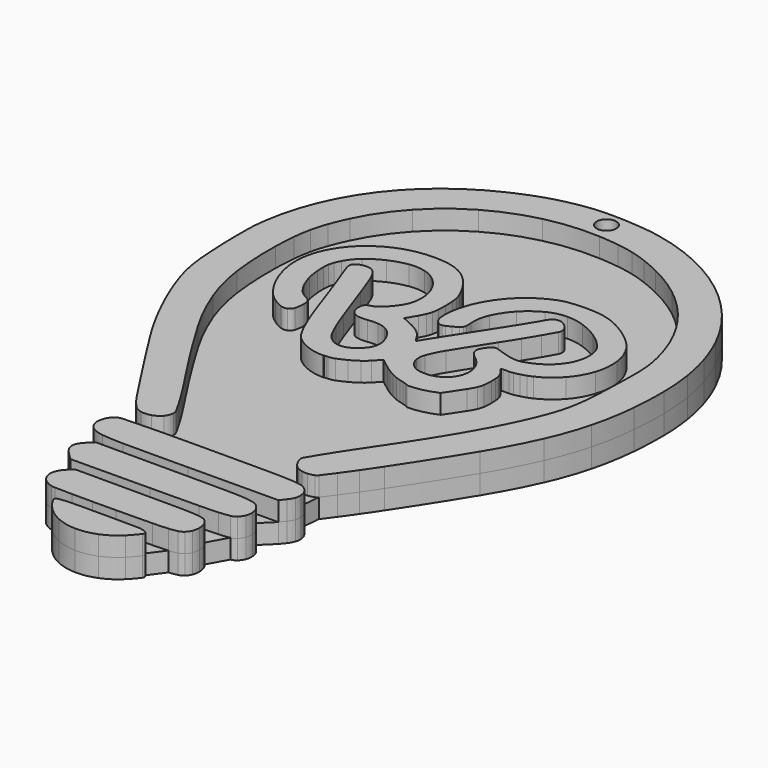
from build123d import *

# Parameters (mm, degrees)
F1_DEPTH = 1
F2_DEPTH = 1
F3_DEPTH = 1
F5_DEPTH = 1
F6_R     = 0.5019925972
F7_DEPTH = 25.4
F8_DEPTH = 25.4


# Not quite as in the source:
# - ends of sketch curves that miss each other by under 0.0002 mm in the source are joined


with BuildPart() as f1:
    # F0 (on Top) → F1 (new body)
    with BuildSketch(Plane.XY):
        with BuildLine():
            ThreePointArc((-17.9502112674, 20.1905372115), (-18.3634901212, 20.17199212), (-18.7749132586, 20.1286985466))
            ThreePointArc((-18.7749132586, 20.1286985466), (-19.224494759, 20.0595403318), (-19.6713317355, 19.9744339226))
            ThreePointArc((-19.6713317355, 19.9744339226), (-20.0910308395, 19.8775167768), (-20.5063033077, 19.7631093914))
            ThreePointArc((-20.5063033077, 19.7631093914), (-20.9225653479, 19.6296074435), (-21.3329820378, 19.4790916774))
            ThreePointArc((-21.3329820378, 19.4790916774), (-21.771878013, 19.2995942783), (-22.2047550163, 19.1060316419))
            ThreePointArc((-22.2047550163, 19.1060316419), (-23.3868306494, 18.4681698853), (-24.4868060277, 17.6973102477))
            ThreePointArc((-24.4868060277, 17.6973102477), (-25.458310568, 16.8232236084), (-26.3119002731, 15.8336615235))
            ThreePointArc((-26.3119002731, 15.8336615235), (-27.0260614158, 14.754599548), (-27.5968162311, 13.5932900052))
            ThreePointArc((-27.5968162311, 13.5932900052), (-28.0217947234, 12.3564369878), (-28.290730911, 11.0765598716))
            ThreePointArc((-28.290730911, 11.0765598716), (-28.3518266489, 10.5349637529), (-28.3772233698, 9.9905245462))
            ThreePointArc((-28.3772233698, 9.9905245462), (-28.3786705105, 9.2162781337), (-28.3617129243, 8.4422160938))
            ThreePointArc((-28.3617129243, 8.4422160938), (-28.3264945975, 7.6708387012), (-28.2730301694, 6.9005108699))
            ThreePointArc((-28.2730301694, 6.9005108699), (-28.2114845251, 6.3689362685), (-28.1138158878, 5.8427991559))
            ThreePointArc((-28.1138158878, 5.8427991559), (-27.9986786379, 5.3819208607), (-27.8587172922, 4.9279646814))
            ThreePointArc((-27.8587172922, 4.9279646814), (-27.6657685186, 4.3851173705), (-27.4562857607, 3.8484336608))
            ThreePointArc((-27.4562857607, 3.8484336608), (-27.2088585243, 3.2660766333), (-26.9448736105, 2.6910358443))
            ThreePointArc((-26.9448736105, 2.6910358443), (-26.6579502393, 2.10889831), (-26.3556944439, 1.5345721271))
            ThreePointArc((-26.3556944439, 1.5345721271), (-25.9845324763, 0.8763908061), (-25.5928089244, 0.2302356257))
            ThreePointArc((-25.5928089244, 0.2302356257), (-24.8884558733, -0.8830741571), (-24.176686144, -1.9916569217))
            ThreePointArc((-24.176686144, -1.9916569217), (-23.4425762443, -3.1214819554), (-22.7037366613, -4.248219734))
            ThreePointArc((-22.7037366613, -4.248219734), (-22.4584579474, -4.5900474479), (-22.1867000659, -4.9112257296))
            ThreePointArc((-22.1867000659, -4.9112257296), (-21.9925982487, -5.0658222025), (-21.7604025915, -5.1533479919))
            ThreePointArc((-21.7604025915, -5.1533479919), (-21.4950450412, -5.1738869828), (-21.2330570593, -5.1269958272))
            ThreePointArc((-21.2330570593, -5.1269958272), (-21.0016294454, -5.0182555931), (-20.8075794463, -4.8517390237))
            ThreePointArc((-20.8075794463, -4.8517390237), (-20.6879609851, -4.6544217335), (-20.6462739343, -4.4274748648))
            ThreePointArc((-20.6462739343, -4.4274748648), (-20.6618091209, -4.3031294773), (-20.7074596912, -4.1864283941))
            ThreePointArc((-20.7074596912, -4.1864283941), (-20.8830586322, -3.869034907), (-21.0638193229, -3.5545524971))
            ThreePointArc((-21.0638193229, -3.5545524971), (-21.3167947694, -3.1319751413), (-21.5778205058, -2.7143224582))
            ThreePointArc((-21.5778205058, -2.7143224582), (-21.9428780671, -2.1472824157), (-22.3122717364, -1.583057505))
            ThreePointArc((-22.3122717364, -1.583057505), (-23.4947158254, 0.2558200872), (-24.632532171, 2.1226405896))
            ThreePointArc((-24.632532171, 2.1226405896), (-25.2953575835, 3.3575901804), (-25.8503409212, 4.6446144643))
            ThreePointArc((-25.8503409212, 4.6446144643), (-26.2014029788, 5.7555556977), (-26.4208094566, 6.8998003401))
            ThreePointArc((-26.4208094566, 6.8998003401), (-26.5428093926, 8.2245001035), (-26.5604218118, 9.5546892794))
            ThreePointArc((-26.5604218118, 9.5546892794), (-26.5364807398, 10.1235242852), (-26.4943471316, 10.691301703))
            ThreePointArc((-26.4943471316, 10.691301703), (-26.4395151988, 11.1387888814), (-26.3563103062, 11.5818783349))
            ThreePointArc((-26.3563103062, 11.5818783349), (-26.2492475876, 11.9983278621), (-26.1140010788, 12.4064957402))
            ThreePointArc((-26.1140010788, 12.4064957402), (-25.9300178462, 12.872850087), (-25.7260306164, 13.3308079644))
            ThreePointArc((-25.7260306164, 13.3308079644), (-25.0682865859, 14.4856081741), (-24.2410604595, 15.5257464587))
            ThreePointArc((-24.2410604595, 15.5257464587), (-23.2564572236, 16.4374825838), (-22.1468568523, 17.1921303911))
            ThreePointArc((-22.1468568523, 17.1921303911), (-20.9199042704, 17.7829990406), (-19.6195737136, 18.1875714769))
            ThreePointArc((-19.6195737136, 18.1875714769), (-18.2551726858, 18.4043444664), (-16.8738484576, 18.427236446))
            ThreePointArc((-16.8738484576, 18.427236446), (-16.3558133922, 18.3898613357), (-15.8394704132, 18.3337617985))
            ThreePointArc((-15.8394704132, 18.3337617985), (-15.4071451672, 18.265581189), (-14.9797041057, 18.1715181614))
            ThreePointArc((-14.9797041057, 18.1715181614), (-14.5639071192, 18.0531562436), (-14.1561344773, 17.9095660394))
            ThreePointArc((-14.1561344773, 17.9095660394), (-13.691223119, 17.7191260506), (-13.2341241714, 17.5106302106))
            ThreePointArc((-13.2341241714, 17.5106302106), (-12.3653935285, 17.0358262662), (-11.551403176, 16.4723092534))
            ThreePointArc((-11.551403176, 16.4723092534), (-10.8163066448, 15.8356432686), (-10.1563485119, 15.1213843923))
            ThreePointArc((-10.1563485119, 15.1213843923), (-9.5833931065, 14.3427838878), (-9.1009456608, 13.5050839997))
            ThreePointArc((-9.1009456608, 13.5050839997), (-8.7111135105, 12.6127023646), (-8.4210891125, 11.6830788108))
            ThreePointArc((-8.4210891125, 11.6830788108), (-8.3499282658, 11.3773801105), (-8.2904187018, 11.069201312))
            ThreePointArc((-8.2904187018, 11.069201312), (-8.2505726442, 10.7949263026), (-8.2258682736, 10.5188752504))
            ThreePointArc((-8.2258682736, 10.5188752504), (-8.2106815692, 10.1698136273), (-8.208255481, 9.8204302174))
            ThreePointArc((-8.208255481, 9.8204302174), (-8.2174724496, 9.218343122), (-8.2314840351, 8.6163485221))
            ThreePointArc((-8.2314840351, 8.6163485221), (-8.2627178486, 7.8250882579), (-8.3132462912, 7.0348254952))
            ThreePointArc((-8.3132462912, 7.0348254952), (-8.3741711163, 6.4891627737), (-8.4732637556, 5.9491254696))
            ThreePointArc((-8.4732637556, 5.9491254696), (-8.6050716645, 5.4433168926), (-8.7752053402, 4.9490799305))
            ThreePointArc((-8.7752053402, 4.9490799305), (-9.0362334168, 4.3079851932), (-9.3186867702, 3.6760372353))
            ThreePointArc((-9.3186867702, 3.6760372353), (-9.6065938335, 3.0821426356), (-9.911303007, 2.4966910222))
            ThreePointArc((-9.911303007, 2.4966910222), (-10.2580358618, 1.8698980185), (-10.6186595079, 1.2509927525))
            ThreePointArc((-10.6186595079, 1.2509927525), (-11.0579377694, 0.5311419383), (-11.5103502521, -0.1805276))
            ThreePointArc((-11.5103502521, -0.1805276), (-12.0888850012, -1.0632431632), (-12.6757423009, -1.9404476605))
            ThreePointArc((-12.6757423009, -1.9404476605), (-12.9583861058, -2.3626562824), (-13.2372773953, -2.7873529847))
            ThreePointArc((-13.2372773953, -2.7873529847), (-13.4764480084, -3.1605152631), (-13.7106285009, -3.5368291824))
            ThreePointArc((-13.7106285009, -3.5368291824), (-13.9061252823, -3.8578955887), (-14.0996515762, -4.1801535635))
            ThreePointArc((-14.0996515762, -4.1801535635), (-14.1305243141, -4.2525056428), (-14.1410677886, -4.330459369))
            ThreePointArc((-14.1410677886, -4.330459369), (-14.136814421, -4.384573461), (-14.1241587812, -4.4373585051))
            ThreePointArc((-14.1241587812, -4.4373585051), (-14.0985298369, -4.5090898965), (-14.0687298925, -4.5791912412))
            ThreePointArc((-14.0687298925, -4.5791912412), (-14.0310161494, -4.6553868796), (-13.9890594649, -4.7293310363))
            ThreePointArc((-13.9890594649, -4.7293310363), (-13.9440150737, -4.7988541618), (-13.8948110097, -4.8654981599))
            ThreePointArc((-13.8948110097, -4.8654981599), (-13.7958043795, -4.9704715202), (-13.6796661551, -5.0561081381))
            ThreePointArc((-13.6796661551, -5.0561081381), (-13.5477300602, -5.1217234895), (-13.4066609137, -5.1642911396))
            ThreePointArc((-13.4066609137, -5.1642911396), (-13.2523353427, -5.1844919687), (-13.0967508594, -5.1802582181))
            ThreePointArc((-13.0967508594, -5.1802582181), (-12.93333449, -5.152035364), (-12.7749684407, -5.1028252808))
            ThreePointArc((-12.7749684407, -5.1028252808), (-12.7089611664, -5.0661476233), (-12.6557430836, -5.0125748164))
            ThreePointArc((-12.6557430836, -5.0125748164), (-12.4222506711, -4.6980485788), (-12.1904658417, -4.3822618566))
            ThreePointArc((-12.1904658417, -4.3822618566), (-11.9215166403, -4.0088043002), (-11.6573227381, -3.6319677296))
            ThreePointArc((-11.6573227381, -3.6319677296), (-11.3579976409, -3.1953251525), (-11.0623289494, -2.756198429))
            ThreePointArc((-11.0623289494, -2.756198429), (-9.9437999973, -1.0413027953), (-8.8613978381, 0.6966211426))
            ThreePointArc((-8.8613978381, 0.6966211426), (-8.1674972259, 1.9207371434), (-7.5504456099, 3.1853340552))
            ThreePointArc((-7.5504456099, 3.1853340552), (-7.1279292565, 4.2408119671), (-6.7961429441, 5.3282270348))
            ThreePointArc((-6.7961429441, 5.3282270348), (-6.5547506439, 6.4475393169), (-6.4068045732, 7.5829873263))
            ThreePointArc((-6.4068045732, 7.5829873263), (-6.3472961211, 8.5200736827), (-6.3341898558, 9.4589561704))
            ThreePointArc((-6.3341898558, 9.4589561704), (-6.3725818463, 10.2912769893), (-6.469629863, 11.1188116267))
            ThreePointArc((-6.469629863, 11.1188116267), (-6.6179691767, 11.8900912049), (-6.824358884, 12.6479038629))
            ThreePointArc((-6.824358884, 12.6479038629), (-7.0902514094, 13.3991570288), (-7.4099774918, 14.1291264712))
            ThreePointArc((-7.4099774918, 14.1291264712), (-8.0003130749, 15.1872156108), (-8.7125810575, 16.1673804157))
            ThreePointArc((-8.7125810575, 16.1673804157), (-9.5488810094, 17.0745910612), (-10.4822885661, 17.8815477532))
            ThreePointArc((-10.4822885661, 17.8815477532), (-11.5100666141, 18.5850841407), (-12.6100568859, 19.1693037661))
            ThreePointArc((-12.6100568859, 19.1693037661), (-13.7671633985, 19.6260977712), (-14.9682166835, 19.9501768616))
            ThreePointArc((-14.9682166835, 19.9501768616), (-15.4116685948, 20.0320551601), (-15.8586287561, 20.0918904851))
            ThreePointArc((-15.8586287561, 20.0918904851), (-16.3856742417, 20.1410277211), (-16.9139807627, 20.173946287))
            ThreePointArc((-16.9139807627, 20.173946287), (-17.431968033, 20.1902352168), (-17.9502112674, 20.1905372115))
        make_face()
        with BuildLine():
            Line((-12.7595410542, -6.1097191234), (-12.6557430836, -5.0125748164))
            ThreePointArc((-12.6557430836, -5.0125748164), (-12.7089611664, -5.0661476233), (-12.774968455, -5.1028252436))
            ThreePointArc((-12.774968455, -5.1028252436), (-12.93333449, -5.152035364), (-13.0967508663, -5.1802581532))
            ThreePointArc((-13.0967508663, -5.1802581532), (-13.2523353427, -5.1844919687), (-13.4066609201, -5.1642911697))
            ThreePointArc((-13.4066609201, -5.1642911697), (-13.5477300602, -5.1217234895), (-13.6796661849, -5.0561081871))
            ThreePointArc((-13.6796661849, -5.0561081871), (-13.7958043795, -4.9704715202), (-13.8948109582, -4.8654981194))
            ThreePointArc((-13.8948109582, -4.8654981194), (-13.9440150737, -4.7988541618), (-13.989059505, -4.7293310606))
            ThreePointArc((-13.989059505, -4.7293310606), (-14.0310161494, -4.6553868796), (-14.0687298833, -4.579191237))
            ThreePointArc((-14.0687298833, -4.579191237), (-14.0985298369, -4.5090898965), (-14.1241587642, -4.4373584996))
            ThreePointArc((-14.1241587642, -4.4373584996), (-14.136814421, -4.384573461), (-14.1410677886, -4.330459369))
            ThreePointArc((-14.1410677886, -4.330459369), (-14.1305243141, -4.2525056428), (-14.0996515333, -4.1801535891))
            ThreePointArc((-14.0996515333, -4.1801535891), (-13.9061252823, -3.8578955887), (-13.7106284858, -3.5368291917))
            ThreePointArc((-13.7106284858, -3.5368291917), (-13.4764480084, -3.1605152631), (-13.2372775028, -2.7873529147))
            ThreePointArc((-13.2372775028, -2.7873529147), (-12.9583861058, -2.3626562824), (-12.6757421792, -1.9404477427))
            ThreePointArc((-12.6757421792, -1.9404477427), (-12.0888850012, -1.0632431632), (-11.5103503639, -0.1805275275))
            ThreePointArc((-11.5103503639, -0.1805275275), (-11.0579377694, 0.5311419383), (-10.6186594858, 1.2509927394))
            ThreePointArc((-10.6186594858, 1.2509927394), (-10.2580358618, 1.8698980185), (-9.9113029971, 2.4966910168))
            ThreePointArc((-9.9113029971, 2.4966910168), (-9.6065938335, 3.0821426356), (-9.3186868058, 3.676037252))
            ThreePointArc((-9.3186868058, 3.676037252), (-9.0362334168, 4.3079851932), (-8.7752053724, 4.949079943))
            ThreePointArc((-8.7752053724, 4.949079943), (-8.6050716645, 5.4433168926), (-8.4732637341, 5.9491254649))
            ThreePointArc((-8.4732637341, 5.9491254649), (-8.3741711163, 6.4891627737), (-8.3132462616, 7.0348254929))
            ThreePointArc((-8.3132462616, 7.0348254929), (-8.2627178486, 7.8250882579), (-8.231483987, 8.6163485208))
            ThreePointArc((-8.231483987, 8.6163485208), (-8.2174724496, 9.218343122), (-8.2082555174, 9.8204302178))
            ThreePointArc((-8.2082555174, 9.8204302178), (-8.2106815692, 10.1698136273), (-8.2258682482, 10.518875252))
            ThreePointArc((-8.2258682482, 10.518875252), (-8.2505726442, 10.7949263026), (-8.290418686, 11.0692013147))
            ThreePointArc((-8.290418686, 11.0692013147), (-8.3499282658, 11.3773801105), (-8.4210892242, 11.6830787826))
            ThreePointArc((-8.4210892242, 11.6830787826), (-8.7111135105, 12.6127023646), (-9.1009455349, 13.5050840632))
            ThreePointArc((-9.1009455349, 13.5050840632), (-9.5833931065, 14.3427838878), (-10.1563485246, 15.1213843818))
            ThreePointArc((-10.1563485246, 15.1213843818), (-10.8163066448, 15.8356432686), (-11.5514032151, 16.4723092029))
            ThreePointArc((-11.5514032151, 16.4723092029), (-12.3653935285, 17.0358262662), (-13.2341241628, 17.5106302286))
            ThreePointArc((-13.2341241628, 17.5106302286), (-13.691223119, 17.7191260506), (-14.1561344293, 17.9095661636))
            ThreePointArc((-14.1561344293, 17.9095661636), (-14.5639071192, 18.0531562436), (-14.9797041367, 18.1715180386))
            ThreePointArc((-14.9797041367, 18.1715180386), (-15.4071451672, 18.265581189), (-15.8394704115, 18.3337618118))
            ThreePointArc((-15.8394704115, 18.3337618118), (-16.3558133922, 18.3898613357), (-16.8738484513, 18.4272365617))
            ThreePointArc((-16.8738484513, 18.4272365617), (-18.2551726858, 18.4043444664), (-19.6195736814, 18.1875713382))
            ThreePointArc((-19.6195736814, 18.1875713382), (-20.9199042704, 17.7829990406), (-22.146856887, 17.1921304514))
            ThreePointArc((-22.146856887, 17.1921304514), (-23.2564572236, 16.4374825838), (-24.2410604706, 15.5257464691))
            ThreePointArc((-24.2410604706, 15.5257464691), (-25.0682865859, 14.4856081741), (-25.7260305345, 13.3308079257))
            ThreePointArc((-25.7260305345, 13.3308079257), (-25.9300178462, 12.872850087), (-26.114001111, 12.4064957521))
            ThreePointArc((-26.114001111, 12.4064957521), (-26.2492475876, 11.9983278621), (-26.3563103228, 11.5818783386))
            ThreePointArc((-26.3563103228, 11.5818783386), (-26.4395151988, 11.1387888814), (-26.494347211, 10.6913017102))
            ThreePointArc((-26.494347211, 10.6913017102), (-26.5364807398, 10.1235242852), (-26.5604217296, 9.5546892773))
            ThreePointArc((-26.5604217296, 9.5546892773), (-26.5428093926, 8.2245001035), (-26.4208093956, 6.8998003482))
            ThreePointArc((-26.4208093956, 6.8998003482), (-26.2014029788, 5.7555556977), (-25.8503410025, 4.6446144333))
            ThreePointArc((-25.8503410025, 4.6446144333), (-25.2953575835, 3.3575901804), (-24.6325321223, 2.1226406185))
            ThreePointArc((-24.6325321223, 2.1226406185), (-23.4947158254, 0.2558200872), (-22.3122717574, -1.5830575189))
            ThreePointArc((-22.3122717574, -1.5830575189), (-21.9428780671, -2.1472824157), (-21.5778205365, -2.7143224778))
            ThreePointArc((-21.5778205365, -2.7143224778), (-21.3167947694, -3.1319751413), (-21.0638192768, -3.5545524701))
            ThreePointArc((-21.0638192768, -3.5545524701), (-20.8830586322, -3.869034907), (-20.707459736, -4.1864284184))
            ThreePointArc((-20.707459736, -4.1864284184), (-20.6618091209, -4.3031294773), (-20.6462739343, -4.4274748648))
            ThreePointArc((-20.6462739343, -4.4274748648), (-20.6879609851, -4.6544217335), (-20.807579427, -4.8517390408))
            ThreePointArc((-20.807579427, -4.8517390408), (-21.0016294454, -5.0182555931), (-21.2330570981, -5.1269957035))
            ThreePointArc((-21.2330570981, -5.1269957035), (-21.4950450412, -5.1738869828), (-21.7604026021, -5.153348043))
            ThreePointArc((-21.7604026021, -5.153348043), (-21.9925982487, -5.0658222025), (-22.186700086, -4.911225748))
            Line((-22.186700086, -4.911225748), (-21.9484925194, -6.0937510862))
            ThreePointArc((-21.9484925194, -6.0937510862), (-21.3806621081, -6.0738039112), (-20.812739607, -6.0566779464))
            ThreePointArc((-20.812739607, -6.0566779464), (-20.0746838132, -6.0396449877), (-19.3365027787, -6.0293864883))
            ThreePointArc((-19.3365027787, -6.0293864883), (-18.3359788407, -6.0219633686), (-17.3354339987, -6.0183202697))
            ThreePointArc((-17.3354339987, -6.0183202697), (-15.8582803767, -6.0169586688), (-14.3811265298, -6.0180490179))
            ThreePointArc((-14.3811265298, -6.0180490179), (-13.8522371738, -6.0250929524), (-13.3236593479, -6.0445621732))
            ThreePointArc((-13.3236593479, -6.0445621732), (-13.0405177514, -6.0677689713), (-12.7595410542, -6.1097191234))
        make_face()
        with BuildLine():
            ThreePointArc((-12.4342512585, -6.2565356216), (-12.5879497455, -6.1633055119), (-12.7595410542, -6.1097191234))
            ThreePointArc((-12.7595410542, -6.1097191234), (-13.0405177514, -6.0677689713), (-13.3236593483, -6.0445621806))
            ThreePointArc((-13.3236593483, -6.0445621806), (-13.8522371738, -6.0250929524), (-14.3811265297, -6.0180489711))
            ThreePointArc((-14.3811265297, -6.0180489711), (-15.8582803767, -6.0169586688), (-17.3354339985, -6.0183203948))
            ThreePointArc((-17.3354339985, -6.0183203948), (-18.3359788407, -6.0219633686), (-19.3365027787, -6.0293864865))
            ThreePointArc((-19.3365027787, -6.0293864865), (-20.0746838132, -6.0396449877), (-20.8127396073, -6.0566779379))
            ThreePointArc((-20.8127396073, -6.0566779379), (-21.3806621081, -6.0738039112), (-21.9484925194, -6.0937510862))
            ThreePointArc((-21.9484925194, -6.0937510862), (-22.0695960289, -6.1109058966), (-22.1846202141, -6.1524965539))
            ThreePointArc((-22.1846202141, -6.1524965539), (-22.2987122753, -6.2243651353), (-22.3939798257, -6.3197914654))
            ThreePointArc((-22.3939798257, -6.3197914654), (-22.4795413041, -6.4462369656), (-22.5445236343, -6.5843909583))
            ThreePointArc((-22.5445236343, -6.5843909583), (-22.5881364348, -6.7329671332), (-22.6085901332, -6.8864552618))
            ThreePointArc((-22.6085901332, -6.8864552618), (-22.6020543481, -7.02657687), (-22.567112884, -7.1624292689))
            ThreePointArc((-22.567112884, -7.1624292689), (-22.4436443735, -7.3748317427), (-22.2557001796, -7.5330602545))
            ThreePointArc((-22.2557001796, -7.5330602545), (-21.9889848141, -7.6534055936), (-21.7032083412, -7.7162696857))
            ThreePointArc((-21.7032083412, -7.7162696857), (-21.1433178177, -7.7637347104), (-20.5816391566, -7.7794638756))
            ThreePointArc((-20.5816391566, -7.7794638756), (-18.9080116029, -7.7760673228), (-17.2344059485, -7.7668564982))
            Line((-17.2344059485, -7.7668564982), (-12.5752691844, -7.733118834))
            Line((-12.5752691844, -7.733118834), (-12.348227747, -7.4526186224))
            ThreePointArc((-12.348227747, -7.4526186224), (-12.2472125262, -7.3041562226), (-12.1721172033, -7.1410432269))
            ThreePointArc((-12.1721172033, -7.1410432269), (-12.1321487757, -6.9800876211), (-12.1266327947, -6.8143355137))
            ThreePointArc((-12.1266327947, -6.8143355137), (-12.1556459353, -6.6564614642), (-12.2183973258, -6.5087176446))
            ThreePointArc((-12.2183973258, -6.5087176446), (-12.313905674, -6.3719969864), (-12.4342512585, -6.2565356216))
        make_face()
        with BuildLine():
            Line((-13.3419479565, -8.4874245585), (-12.5752691844, -7.733118834))
            Line((-12.5752691844, -7.733118834), (-17.234405949, -7.7668564371))
            ThreePointArc((-17.234405949, -7.7668564371), (-18.9080116029, -7.7760673228), (-20.5816391565, -7.7794640034))
            ThreePointArc((-20.5816391565, -7.7794640034), (-21.1433178177, -7.7637347104), (-21.7032083342, -7.716269624))
            ThreePointArc((-21.7032083342, -7.716269624), (-21.9889848141, -7.6534055936), (-22.2557001768, -7.5330602498))
            Line((-22.2557001768, -7.5330602498), (-21.51849542, -8.3866098623))
            Line((-21.51849542, -8.3866098623), (-17.429947099, -8.3866098623))
            ThreePointArc((-17.429947099, -8.3866098623), (-16.1242093709, -8.3878808679), (-14.8184765886, -8.3916928343))
            ThreePointArc((-14.8184765886, -8.3916928343), (-14.3386059788, -8.3997993347), (-13.8591082716, -8.4203776343))
            ThreePointArc((-13.8591082716, -8.4203776343), (-13.5993033368, -8.4444538966), (-13.3419479565, -8.4874245585))
        make_face()
        with BuildLine():
            ThreePointArc((-13.0283340097, -8.6328666314), (-13.1766570441, -8.5418518296), (-13.341947941, -8.4874244828))
            ThreePointArc((-13.341947941, -8.4874244828), (-13.5993033368, -8.4444538966), (-13.8591082745, -8.4203776868))
            ThreePointArc((-13.8591082745, -8.4203776868), (-14.3386059788, -8.3997993347), (-14.8184765886, -8.3916928233))
            ThreePointArc((-14.8184765886, -8.3916928233), (-16.1242093709, -8.3878808679), (-17.429947099, -8.3866098623))
            Line((-17.429947099, -8.3866098623), (-21.51849542, -8.3866098623))
            Line((-21.51849542, -8.3866098623), (-21.810136109, -8.6782504325))
            ThreePointArc((-21.810136109, -8.6782504325), (-21.9266295023, -8.8126614335), (-22.0228413611, -8.9622619206))
            ThreePointArc((-22.0228413611, -8.9622619206), (-22.0730709744, -9.094865574), (-22.0852232202, -9.2361421428))
            ThreePointArc((-22.0852232202, -9.2361421428), (-22.0586249273, -9.3826284256), (-21.9959953272, -9.517695943))
            ThreePointArc((-21.9959953272, -9.517695943), (-21.8816420792, -9.6787432185), (-21.7500103189, -9.8260047846))
            Line((-21.7500103189, -9.8260047846), (-21.3982438031, -10.1777711449))
            Line((-21.3982438031, -10.1777711449), (-17.3067117609, -10.1436104361))
            ThreePointArc((-17.3067117609, -10.1436104361), (-16.0490651571, -10.1317703572), (-14.7914466548, -10.1172489852))
            ThreePointArc((-14.7914466548, -10.1172489852), (-14.2892583743, -10.104972328), (-13.7875011057, -10.0808180786))
            ThreePointArc((-13.7875011057, -10.0808180786), (-13.5125070591, -10.0565511197), (-13.2393092116, -10.0168831356))
            ThreePointArc((-13.2393092116, -10.0168831356), (-13.0927795504, -9.9694320318), (-12.9652244419, -9.8831056863))
            ThreePointArc((-12.9652244419, -9.8831056863), (-12.8505732252, -9.7525833898), (-12.7684448044, -9.5994955127))
            ThreePointArc((-12.7684448044, -9.5994955127), (-12.7209212599, -9.4284869565), (-12.7108577291, -9.2512832874))
            ThreePointArc((-12.7108577291, -9.2512832874), (-12.7387492202, -9.0739816114), (-12.8031881853, -8.9064661259))
            ThreePointArc((-12.8031881853, -8.9064661259), (-12.9009478082, -8.7574764814), (-13.0283340097, -8.6328666314))
        make_face()
        with BuildLine():
            Line((-13.7846181923, -11.0005740311), (-13.2393092323, -10.0168830168))
            ThreePointArc((-13.2393092323, -10.0168830168), (-13.5125070591, -10.0565511197), (-13.7875010984, -10.0808182007))
            ThreePointArc((-13.7875010984, -10.0808182007), (-14.2892583743, -10.104972328), (-14.7914466559, -10.1172488977))
            ThreePointArc((-14.7914466559, -10.1172488977), (-16.0490651571, -10.1317703572), (-17.3067117607, -10.1436104566))
            Line((-17.3067117607, -10.1436104566), (-21.3982438031, -10.1777711449))
            Line((-21.3982438031, -10.1777711449), (-20.6867795657, -10.7629408744))
            Line((-20.6867795657, -10.7629408744), (-17.3545154613, -10.7629408744))
            ThreePointArc((-17.3545154613, -10.7629408744), (-16.309884614, -10.7642617573), (-15.265260444, -10.7682234585))
            ThreePointArc((-15.265260444, -10.7682234585), (-14.8645361047, -10.7764032227), (-14.4642517812, -10.7968816031))
            ThreePointArc((-14.4642517812, -10.7968816031), (-14.2470741563, -10.8204670833), (-14.0326167973, -10.8620656158))
            ThreePointArc((-14.0326167973, -10.8620656158), (-13.8989974914, -10.9140952683), (-13.7846181923, -11.0005740311))
        make_face()
        with BuildLine():
            ThreePointArc((-13.6076584061, -11.2816975183), (-13.6803585574, -11.1312028454), (-13.7846181923, -11.0005740311))
            ThreePointArc((-13.7846181923, -11.0005740311), (-13.8989974914, -10.9140952683), (-14.0326167901, -10.8620655856))
            ThreePointArc((-14.0326167901, -10.8620655856), (-14.2470741563, -10.8204670833), (-14.4642517771, -10.7968815417))
            ThreePointArc((-14.4642517771, -10.7968815417), (-14.8645361047, -10.7764032227), (-15.2652604443, -10.7682235294))
            ThreePointArc((-15.2652604443, -10.7682235294), (-16.309884614, -10.7642617573), (-17.3545154613, -10.7629408744))
            Line((-17.3545154613, -10.7629408744), (-20.6867795657, -10.7629408744))
            Line((-20.6867795657, -10.7629408744), (-20.9784202548, -11.0545814446))
            ThreePointArc((-20.9784202548, -11.0545814446), (-21.1224181988, -11.2398395595), (-21.2162504695, -11.4549011383))
            ThreePointArc((-21.2162504695, -11.4549011383), (-21.246968057, -11.6742494387), (-21.2125379285, -11.8930457218))
            ThreePointArc((-21.2125379285, -11.8930457218), (-21.1146703905, -12.0977828139), (-20.9632832177, -12.2668308917))
            ThreePointArc((-20.9632832177, -12.2668308917), (-20.7587517185, -12.4023464086), (-20.529040267, -12.4885452808))
            ThreePointArc((-20.529040267, -12.4885452808), (-20.4298543607, -12.5074503519), (-20.3291533934, -12.5148369113))
            ThreePointArc((-20.3291533934, -12.5148369113), (-19.8770434038, -12.5212422241), (-19.424916313, -12.5262983638))
            ThreePointArc((-19.424916313, -12.5262983638), (-18.8932453856, -12.5297800994), (-18.3615630775, -12.5299220557))
            ThreePointArc((-18.3615630775, -12.5299220557), (-17.7567699792, -12.5268905058), (-17.1519953843, -12.5212716539))
            ThreePointArc((-17.1519953843, -12.5212716539), (-16.216318628, -12.509126326), (-15.2806840196, -12.494080357))
            ThreePointArc((-15.2806840196, -12.494080357), (-14.8844570042, -12.4811216792), (-14.488800105, -12.4562340686))
            ThreePointArc((-14.488800105, -12.4562340686), (-14.2669871884, -12.4308666406), (-14.0475728102, -12.3896136691))
            ThreePointArc((-14.0475728102, -12.3896136691), (-13.9138067967, -12.3407280377), (-13.7968671666, -12.2594367617))
            ThreePointArc((-13.7968671666, -12.2594367617), (-13.6898569527, -12.1365559799), (-13.6146347725, -11.9920136159))
            ThreePointArc((-13.6146347725, -11.9920136159), (-13.5659620797, -11.8185671107), (-13.5483931878, -11.639279473))
            ThreePointArc((-13.5483931878, -11.639279473), (-13.5624338192, -11.4579042947), (-13.6076584061, -11.2816975183))
        make_face()
        with BuildLine():
            Line((-15.0742861752, -13.2509467162), (-14.488800105, -12.4562340686))
            ThreePointArc((-14.488800105, -12.4562340686), (-14.8844570042, -12.4811216792), (-15.2806840197, -12.4940803504))
            ThreePointArc((-15.2806840197, -12.4940803504), (-16.216318628, -12.509126326), (-17.1519953831, -12.5212717624))
            ThreePointArc((-17.1519953831, -12.5212717624), (-17.7567699792, -12.5268905058), (-18.3615630774, -12.5299220925))
            ThreePointArc((-18.3615630774, -12.5299220925), (-18.8932453856, -12.5297800994), (-19.4249163109, -12.5262981507))
            ThreePointArc((-19.4249163109, -12.5262981507), (-19.8770434038, -12.5212422241), (-20.3291533942, -12.5148369627))
            Line((-20.3291533942, -12.5148369627), (-19.6458088714, -13.2173890301))
            ThreePointArc((-19.6458088714, -13.2173890301), (-19.4686945007, -13.1892745396), (-19.2902806431, -13.17115217))
            ThreePointArc((-19.2902806431, -13.17115217), (-18.9741014073, -13.1530799987), (-18.6575052815, -13.1451550035))
            ThreePointArc((-18.6575052815, -13.1451550035), (-18.003316581, -13.1407427969), (-17.349114655, -13.1392718865))
            ThreePointArc((-17.349114655, -13.1392718865), (-16.4303644579, -13.1423288316), (-15.5116549588, -13.1515008425))
            ThreePointArc((-15.5116549588, -13.1515008425), (-15.2877237827, -13.1781481438), (-15.0742861752, -13.2509467162))
        make_face()
        with BuildLine():
            ThreePointArc((-15.0176609375, -13.4733993202), (-14.993085801, -13.3487104573), (-15.0742861752, -13.2509467162))
            ThreePointArc((-15.0742861752, -13.2509467162), (-15.2877237827, -13.1781481438), (-15.5116549588, -13.1515008434))
            ThreePointArc((-15.5116549588, -13.1515008434), (-16.4303644579, -13.1423288316), (-17.349114655, -13.1392718865))
            ThreePointArc((-17.349114655, -13.1392718865), (-18.003316581, -13.1407427969), (-18.6575052819, -13.1451549694))
            ThreePointArc((-18.6575052819, -13.1451549694), (-18.9741014073, -13.1530799987), (-19.2902806424, -13.1711521796))
            ThreePointArc((-19.2902806424, -13.1711521796), (-19.4686945007, -13.1892745396), (-19.6458088714, -13.2173890301))
            ThreePointArc((-19.6458088714, -13.2173890301), (-19.702943818, -13.2510067845), (-19.7254456671, -13.3133623717))
            ThreePointArc((-19.7254456671, -13.3133623717), (-19.7196797365, -13.3615010274), (-19.7027082051, -13.406916259))
            ThreePointArc((-19.7027082051, -13.406916259), (-19.6591783776, -13.4869936976), (-19.6123124168, -13.5651654581))
            ThreePointArc((-19.6123124168, -13.5651654581), (-19.551999677, -13.6566361478), (-19.4877605417, -13.7453933833))
            ThreePointArc((-19.4877605417, -13.7453933833), (-19.4156679994, -13.8370770363), (-19.3403110155, -13.9260969893))
            ThreePointArc((-19.3403110155, -13.9260969893), (-18.9467289177, -14.29001939), (-18.4864792254, -14.5648222342))
            ThreePointArc((-18.4864792254, -14.5648222342), (-17.9784890862, -14.73932283), (-17.4454951938, -14.8058204436))
            ThreePointArc((-17.4454951938, -14.8058204436), (-16.9052872238, -14.7617395406), (-16.3852595507, -14.6089684288))
            ThreePointArc((-16.3852595507, -14.6089684288), (-15.9015134595, -14.3527492552), (-15.4777539931, -14.0062143427))
            ThreePointArc((-15.4777539931, -14.0062143427), (-15.2378679126, -13.7483034189), (-15.0176609375, -13.4733993202))
        make_face()
    extrude(amount=-F1_DEPTH)

    # F6 (on Top) → F8 (cut)
    with BuildSketch(Plane.XY):
        with Locations((-17.2685887665, 19.3878244609)):
            Circle(F6_R)
    extrude(amount=-F8_DEPTH, mode=Mode.SUBTRACT)


with BuildPart() as f2:
    # F0 (on Top) → F2 (new body)
    with BuildSketch(Plane.XY):
        with BuildLine():
            ThreePointArc((-17.9502112674, 20.1905372115), (-18.3634901212, 20.17199212), (-18.7749132586, 20.1286985466))
            ThreePointArc((-18.7749132586, 20.1286985466), (-19.224494759, 20.0595403318), (-19.6713317355, 19.9744339226))
            ThreePointArc((-19.6713317355, 19.9744339226), (-20.0910308395, 19.8775167768), (-20.5063033077, 19.7631093914))
            ThreePointArc((-20.5063033077, 19.7631093914), (-20.9225653479, 19.6296074435), (-21.3329820378, 19.4790916774))
            ThreePointArc((-21.3329820378, 19.4790916774), (-21.771878013, 19.2995942783), (-22.2047550163, 19.1060316419))
            ThreePointArc((-22.2047550163, 19.1060316419), (-23.3868306494, 18.4681698853), (-24.4868060277, 17.6973102477))
            ThreePointArc((-24.4868060277, 17.6973102477), (-25.458310568, 16.8232236084), (-26.3119002731, 15.8336615235))
            ThreePointArc((-26.3119002731, 15.8336615235), (-27.0260614158, 14.754599548), (-27.5968162311, 13.5932900052))
            ThreePointArc((-27.5968162311, 13.5932900052), (-28.0217947234, 12.3564369878), (-28.290730911, 11.0765598716))
            ThreePointArc((-28.290730911, 11.0765598716), (-28.3518266489, 10.5349637529), (-28.3772233698, 9.9905245462))
            ThreePointArc((-28.3772233698, 9.9905245462), (-28.3786705105, 9.2162781337), (-28.3617129243, 8.4422160938))
            ThreePointArc((-28.3617129243, 8.4422160938), (-28.3264945975, 7.6708387012), (-28.2730301694, 6.9005108699))
            ThreePointArc((-28.2730301694, 6.9005108699), (-28.2114845251, 6.3689362685), (-28.1138158878, 5.8427991559))
            ThreePointArc((-28.1138158878, 5.8427991559), (-27.9986786379, 5.3819208607), (-27.8587172922, 4.9279646814))
            ThreePointArc((-27.8587172922, 4.9279646814), (-27.6657685186, 4.3851173705), (-27.4562857607, 3.8484336608))
            ThreePointArc((-27.4562857607, 3.8484336608), (-27.2088585243, 3.2660766333), (-26.9448736105, 2.6910358443))
            ThreePointArc((-26.9448736105, 2.6910358443), (-26.6579502393, 2.10889831), (-26.3556944439, 1.5345721271))
            ThreePointArc((-26.3556944439, 1.5345721271), (-25.9845324763, 0.8763908061), (-25.5928089244, 0.2302356257))
            ThreePointArc((-25.5928089244, 0.2302356257), (-24.8884558733, -0.8830741571), (-24.176686144, -1.9916569217))
            ThreePointArc((-24.176686144, -1.9916569217), (-23.4425762443, -3.1214819554), (-22.7037366613, -4.248219734))
            ThreePointArc((-22.7037366613, -4.248219734), (-22.4584579474, -4.5900474479), (-22.1867000659, -4.9112257296))
            ThreePointArc((-22.1867000659, -4.9112257296), (-21.9925982487, -5.0658222025), (-21.7604025915, -5.1533479919))
            ThreePointArc((-21.7604025915, -5.1533479919), (-21.4950450412, -5.1738869828), (-21.2330570593, -5.1269958272))
            ThreePointArc((-21.2330570593, -5.1269958272), (-21.0016294454, -5.0182555931), (-20.8075794463, -4.8517390237))
            ThreePointArc((-20.8075794463, -4.8517390237), (-20.6879609851, -4.6544217335), (-20.6462739343, -4.4274748648))
            ThreePointArc((-20.6462739343, -4.4274748648), (-20.6618091209, -4.3031294773), (-20.7074596912, -4.1864283941))
            ThreePointArc((-20.7074596912, -4.1864283941), (-20.8830586322, -3.869034907), (-21.0638193229, -3.5545524971))
            ThreePointArc((-21.0638193229, -3.5545524971), (-21.3167947694, -3.1319751413), (-21.5778205058, -2.7143224582))
            ThreePointArc((-21.5778205058, -2.7143224582), (-21.9428780671, -2.1472824157), (-22.3122717364, -1.583057505))
            ThreePointArc((-22.3122717364, -1.583057505), (-23.4947158254, 0.2558200872), (-24.632532171, 2.1226405896))
            ThreePointArc((-24.632532171, 2.1226405896), (-25.2953575835, 3.3575901804), (-25.8503409212, 4.6446144643))
            ThreePointArc((-25.8503409212, 4.6446144643), (-26.2014029788, 5.7555556977), (-26.4208094566, 6.8998003401))
            ThreePointArc((-26.4208094566, 6.8998003401), (-26.5428093926, 8.2245001035), (-26.5604218118, 9.5546892794))
            ThreePointArc((-26.5604218118, 9.5546892794), (-26.5364807398, 10.1235242852), (-26.4943471316, 10.691301703))
            ThreePointArc((-26.4943471316, 10.691301703), (-26.4395151988, 11.1387888814), (-26.3563103062, 11.5818783349))
            ThreePointArc((-26.3563103062, 11.5818783349), (-26.2492475876, 11.9983278621), (-26.1140010788, 12.4064957402))
            ThreePointArc((-26.1140010788, 12.4064957402), (-25.9300178462, 12.872850087), (-25.7260306164, 13.3308079644))
            ThreePointArc((-25.7260306164, 13.3308079644), (-25.0682865859, 14.4856081741), (-24.2410604595, 15.5257464587))
            ThreePointArc((-24.2410604595, 15.5257464587), (-23.2564572236, 16.4374825838), (-22.1468568523, 17.1921303911))
            ThreePointArc((-22.1468568523, 17.1921303911), (-20.9199042704, 17.7829990406), (-19.6195737136, 18.1875714769))
            ThreePointArc((-19.6195737136, 18.1875714769), (-18.2551726858, 18.4043444664), (-16.8738484576, 18.427236446))
            ThreePointArc((-16.8738484576, 18.427236446), (-16.3558133922, 18.3898613357), (-15.8394704132, 18.3337617985))
            ThreePointArc((-15.8394704132, 18.3337617985), (-15.4071451672, 18.265581189), (-14.9797041057, 18.1715181614))
            ThreePointArc((-14.9797041057, 18.1715181614), (-14.5639071192, 18.0531562436), (-14.1561344773, 17.9095660394))
            ThreePointArc((-14.1561344773, 17.9095660394), (-13.691223119, 17.7191260506), (-13.2341241714, 17.5106302106))
            ThreePointArc((-13.2341241714, 17.5106302106), (-12.3653935285, 17.0358262662), (-11.551403176, 16.4723092534))
            ThreePointArc((-11.551403176, 16.4723092534), (-10.8163066448, 15.8356432686), (-10.1563485119, 15.1213843923))
            ThreePointArc((-10.1563485119, 15.1213843923), (-9.5833931065, 14.3427838878), (-9.1009456608, 13.5050839997))
            ThreePointArc((-9.1009456608, 13.5050839997), (-8.7111135105, 12.6127023646), (-8.4210891125, 11.6830788108))
            ThreePointArc((-8.4210891125, 11.6830788108), (-8.3499282658, 11.3773801105), (-8.2904187018, 11.069201312))
            ThreePointArc((-8.2904187018, 11.069201312), (-8.2505726442, 10.7949263026), (-8.2258682736, 10.5188752504))
            ThreePointArc((-8.2258682736, 10.5188752504), (-8.2106815692, 10.1698136273), (-8.208255481, 9.8204302174))
            ThreePointArc((-8.208255481, 9.8204302174), (-8.2174724496, 9.218343122), (-8.2314840351, 8.6163485221))
            ThreePointArc((-8.2314840351, 8.6163485221), (-8.2627178486, 7.8250882579), (-8.3132462912, 7.0348254952))
            ThreePointArc((-8.3132462912, 7.0348254952), (-8.3741711163, 6.4891627737), (-8.4732637556, 5.9491254696))
            ThreePointArc((-8.4732637556, 5.9491254696), (-8.6050716645, 5.4433168926), (-8.7752053402, 4.9490799305))
            ThreePointArc((-8.7752053402, 4.9490799305), (-9.0362334168, 4.3079851932), (-9.3186867702, 3.6760372353))
            ThreePointArc((-9.3186867702, 3.6760372353), (-9.6065938335, 3.0821426356), (-9.911303007, 2.4966910222))
            ThreePointArc((-9.911303007, 2.4966910222), (-10.2580358618, 1.8698980185), (-10.6186595079, 1.2509927525))
            ThreePointArc((-10.6186595079, 1.2509927525), (-11.0579377694, 0.5311419383), (-11.5103502521, -0.1805276))
            ThreePointArc((-11.5103502521, -0.1805276), (-12.0888850012, -1.0632431632), (-12.6757423009, -1.9404476605))
            ThreePointArc((-12.6757423009, -1.9404476605), (-12.9583861058, -2.3626562824), (-13.2372773953, -2.7873529847))
            ThreePointArc((-13.2372773953, -2.7873529847), (-13.4764480084, -3.1605152631), (-13.7106285009, -3.5368291824))
            ThreePointArc((-13.7106285009, -3.5368291824), (-13.9061252823, -3.8578955887), (-14.0996515762, -4.1801535635))
            ThreePointArc((-14.0996515762, -4.1801535635), (-14.1305243141, -4.2525056428), (-14.1410677886, -4.330459369))
            ThreePointArc((-14.1410677886, -4.330459369), (-14.136814421, -4.384573461), (-14.1241587812, -4.4373585051))
            ThreePointArc((-14.1241587812, -4.4373585051), (-14.0985298369, -4.5090898965), (-14.0687298925, -4.5791912412))
            ThreePointArc((-14.0687298925, -4.5791912412), (-14.0310161494, -4.6553868796), (-13.9890594649, -4.7293310363))
            ThreePointArc((-13.9890594649, -4.7293310363), (-13.9440150737, -4.7988541618), (-13.8948110097, -4.8654981599))
            ThreePointArc((-13.8948110097, -4.8654981599), (-13.7958043795, -4.9704715202), (-13.6796661551, -5.0561081381))
            ThreePointArc((-13.6796661551, -5.0561081381), (-13.5477300602, -5.1217234895), (-13.4066609137, -5.1642911396))
            ThreePointArc((-13.4066609137, -5.1642911396), (-13.2523353427, -5.1844919687), (-13.0967508594, -5.1802582181))
            ThreePointArc((-13.0967508594, -5.1802582181), (-12.93333449, -5.152035364), (-12.7749684407, -5.1028252808))
            ThreePointArc((-12.7749684407, -5.1028252808), (-12.7089611664, -5.0661476233), (-12.6557430836, -5.0125748164))
            ThreePointArc((-12.6557430836, -5.0125748164), (-12.4222506711, -4.6980485788), (-12.1904658417, -4.3822618566))
            ThreePointArc((-12.1904658417, -4.3822618566), (-11.9215166403, -4.0088043002), (-11.6573227381, -3.6319677296))
            ThreePointArc((-11.6573227381, -3.6319677296), (-11.3579976409, -3.1953251525), (-11.0623289494, -2.756198429))
            ThreePointArc((-11.0623289494, -2.756198429), (-9.9437999973, -1.0413027953), (-8.8613978381, 0.6966211426))
            ThreePointArc((-8.8613978381, 0.6966211426), (-8.1674972259, 1.9207371434), (-7.5504456099, 3.1853340552))
            ThreePointArc((-7.5504456099, 3.1853340552), (-7.1279292565, 4.2408119671), (-6.7961429441, 5.3282270348))
            ThreePointArc((-6.7961429441, 5.3282270348), (-6.5547506439, 6.4475393169), (-6.4068045732, 7.5829873263))
            ThreePointArc((-6.4068045732, 7.5829873263), (-6.3472961211, 8.5200736827), (-6.3341898558, 9.4589561704))
            ThreePointArc((-6.3341898558, 9.4589561704), (-6.3725818463, 10.2912769893), (-6.469629863, 11.1188116267))
            ThreePointArc((-6.469629863, 11.1188116267), (-6.6179691767, 11.8900912049), (-6.824358884, 12.6479038629))
            ThreePointArc((-6.824358884, 12.6479038629), (-7.0902514094, 13.3991570288), (-7.4099774918, 14.1291264712))
            ThreePointArc((-7.4099774918, 14.1291264712), (-8.0003130749, 15.1872156108), (-8.7125810575, 16.1673804157))
            ThreePointArc((-8.7125810575, 16.1673804157), (-9.5488810094, 17.0745910612), (-10.4822885661, 17.8815477532))
            ThreePointArc((-10.4822885661, 17.8815477532), (-11.5100666141, 18.5850841407), (-12.6100568859, 19.1693037661))
            ThreePointArc((-12.6100568859, 19.1693037661), (-13.7671633985, 19.6260977712), (-14.9682166835, 19.9501768616))
            ThreePointArc((-14.9682166835, 19.9501768616), (-15.4116685948, 20.0320551601), (-15.8586287561, 20.0918904851))
            ThreePointArc((-15.8586287561, 20.0918904851), (-16.3856742417, 20.1410277211), (-16.9139807627, 20.173946287))
            ThreePointArc((-16.9139807627, 20.173946287), (-17.431968033, 20.1902352168), (-17.9502112674, 20.1905372115))
        make_face()
    extrude(amount=F2_DEPTH)

    # F6 (on Top) → F7 (cut)
    with BuildSketch(Plane.XY):
        with Locations((-17.2685887665, 19.3878244609)):
            Circle(F6_R)
    extrude(amount=F7_DEPTH, mode=Mode.SUBTRACT)


with BuildPart() as f3:
    # F0 (on Top) → F3 (new body)
    with BuildSketch(Plane.XY):
        with BuildLine():
            ThreePointArc((-12.4342512585, -6.2565356216), (-12.5879497455, -6.1633055119), (-12.7595410542, -6.1097191234))
            ThreePointArc((-12.7595410542, -6.1097191234), (-13.0405177514, -6.0677689713), (-13.3236593483, -6.0445621806))
            ThreePointArc((-13.3236593483, -6.0445621806), (-13.8522371738, -6.0250929524), (-14.3811265297, -6.0180489711))
            ThreePointArc((-14.3811265297, -6.0180489711), (-15.8582803767, -6.0169586688), (-17.3354339985, -6.0183203948))
            ThreePointArc((-17.3354339985, -6.0183203948), (-18.3359788407, -6.0219633686), (-19.3365027787, -6.0293864865))
            ThreePointArc((-19.3365027787, -6.0293864865), (-20.0746838132, -6.0396449877), (-20.8127396073, -6.0566779379))
            ThreePointArc((-20.8127396073, -6.0566779379), (-21.3806621081, -6.0738039112), (-21.9484925194, -6.0937510862))
            ThreePointArc((-21.9484925194, -6.0937510862), (-22.0695960289, -6.1109058966), (-22.1846202141, -6.1524965539))
            ThreePointArc((-22.1846202141, -6.1524965539), (-22.2987122753, -6.2243651353), (-22.3939798257, -6.3197914654))
            ThreePointArc((-22.3939798257, -6.3197914654), (-22.4795413041, -6.4462369656), (-22.5445236343, -6.5843909583))
            ThreePointArc((-22.5445236343, -6.5843909583), (-22.5881364348, -6.7329671332), (-22.6085901332, -6.8864552618))
            ThreePointArc((-22.6085901332, -6.8864552618), (-22.6020543481, -7.02657687), (-22.567112884, -7.1624292689))
            ThreePointArc((-22.567112884, -7.1624292689), (-22.4436443735, -7.3748317427), (-22.2557001796, -7.5330602545))
            ThreePointArc((-22.2557001796, -7.5330602545), (-21.9889848141, -7.6534055936), (-21.7032083412, -7.7162696857))
            ThreePointArc((-21.7032083412, -7.7162696857), (-21.1433178177, -7.7637347104), (-20.5816391566, -7.7794638756))
            ThreePointArc((-20.5816391566, -7.7794638756), (-18.9080116029, -7.7760673228), (-17.2344059485, -7.7668564982))
            Line((-17.2344059485, -7.7668564982), (-12.5752691844, -7.733118834))
            Line((-12.5752691844, -7.733118834), (-12.348227747, -7.4526186224))
            ThreePointArc((-12.348227747, -7.4526186224), (-12.2472125262, -7.3041562226), (-12.1721172033, -7.1410432269))
            ThreePointArc((-12.1721172033, -7.1410432269), (-12.1321487757, -6.9800876211), (-12.1266327947, -6.8143355137))
            ThreePointArc((-12.1266327947, -6.8143355137), (-12.1556459353, -6.6564614642), (-12.2183973258, -6.5087176446))
            ThreePointArc((-12.2183973258, -6.5087176446), (-12.313905674, -6.3719969864), (-12.4342512585, -6.2565356216))
        make_face()
    extrude(amount=F3_DEPTH)


with BuildPart() as f3b:
    # F0 (on Top) → F3, piece 2 (new body)
    with BuildSketch(Plane.XY):
        with BuildLine():
            ThreePointArc((-13.0283340097, -8.6328666314), (-13.1766570441, -8.5418518296), (-13.341947941, -8.4874244828))
            ThreePointArc((-13.341947941, -8.4874244828), (-13.5993033368, -8.4444538966), (-13.8591082745, -8.4203776868))
            ThreePointArc((-13.8591082745, -8.4203776868), (-14.3386059788, -8.3997993347), (-14.8184765886, -8.3916928233))
            ThreePointArc((-14.8184765886, -8.3916928233), (-16.1242093709, -8.3878808679), (-17.429947099, -8.3866098623))
            Line((-17.429947099, -8.3866098623), (-21.51849542, -8.3866098623))
            Line((-21.51849542, -8.3866098623), (-21.810136109, -8.6782504325))
            ThreePointArc((-21.810136109, -8.6782504325), (-21.9266295023, -8.8126614335), (-22.0228413611, -8.9622619206))
            ThreePointArc((-22.0228413611, -8.9622619206), (-22.0730709744, -9.094865574), (-22.0852232202, -9.2361421428))
            ThreePointArc((-22.0852232202, -9.2361421428), (-22.0586249273, -9.3826284256), (-21.9959953272, -9.517695943))
            ThreePointArc((-21.9959953272, -9.517695943), (-21.8816420792, -9.6787432185), (-21.7500103189, -9.8260047846))
            Line((-21.7500103189, -9.8260047846), (-21.3982438031, -10.1777711449))
            Line((-21.3982438031, -10.1777711449), (-17.3067117609, -10.1436104361))
            ThreePointArc((-17.3067117609, -10.1436104361), (-16.0490651571, -10.1317703572), (-14.7914466548, -10.1172489852))
            ThreePointArc((-14.7914466548, -10.1172489852), (-14.2892583743, -10.104972328), (-13.7875011057, -10.0808180786))
            ThreePointArc((-13.7875011057, -10.0808180786), (-13.5125070591, -10.0565511197), (-13.2393092116, -10.0168831356))
            ThreePointArc((-13.2393092116, -10.0168831356), (-13.0927795504, -9.9694320318), (-12.9652244419, -9.8831056863))
            ThreePointArc((-12.9652244419, -9.8831056863), (-12.8505732252, -9.7525833898), (-12.7684448044, -9.5994955127))
            ThreePointArc((-12.7684448044, -9.5994955127), (-12.7209212599, -9.4284869565), (-12.7108577291, -9.2512832874))
            ThreePointArc((-12.7108577291, -9.2512832874), (-12.7387492202, -9.0739816114), (-12.8031881853, -8.9064661259))
            ThreePointArc((-12.8031881853, -8.9064661259), (-12.9009478082, -8.7574764814), (-13.0283340097, -8.6328666314))
        make_face()
    extrude(amount=F3_DEPTH)


with BuildPart() as f3c:
    # F0 (on Top) → F3, piece 3 (new body)
    with BuildSketch(Plane.XY):
        with BuildLine():
            ThreePointArc((-13.6076584061, -11.2816975183), (-13.6803585574, -11.1312028454), (-13.7846181923, -11.0005740311))
            ThreePointArc((-13.7846181923, -11.0005740311), (-13.8989974914, -10.9140952683), (-14.0326167901, -10.8620655856))
            ThreePointArc((-14.0326167901, -10.8620655856), (-14.2470741563, -10.8204670833), (-14.4642517771, -10.7968815417))
            ThreePointArc((-14.4642517771, -10.7968815417), (-14.8645361047, -10.7764032227), (-15.2652604443, -10.7682235294))
            ThreePointArc((-15.2652604443, -10.7682235294), (-16.309884614, -10.7642617573), (-17.3545154613, -10.7629408744))
            Line((-17.3545154613, -10.7629408744), (-20.6867795657, -10.7629408744))
            Line((-20.6867795657, -10.7629408744), (-20.9784202548, -11.0545814446))
            ThreePointArc((-20.9784202548, -11.0545814446), (-21.1224181988, -11.2398395595), (-21.2162504695, -11.4549011383))
            ThreePointArc((-21.2162504695, -11.4549011383), (-21.246968057, -11.6742494387), (-21.2125379285, -11.8930457218))
            ThreePointArc((-21.2125379285, -11.8930457218), (-21.1146703905, -12.0977828139), (-20.9632832177, -12.2668308917))
            ThreePointArc((-20.9632832177, -12.2668308917), (-20.7587517185, -12.4023464086), (-20.529040267, -12.4885452808))
            ThreePointArc((-20.529040267, -12.4885452808), (-20.4298543607, -12.5074503519), (-20.3291533934, -12.5148369113))
            ThreePointArc((-20.3291533934, -12.5148369113), (-19.8770434038, -12.5212422241), (-19.424916313, -12.5262983638))
            ThreePointArc((-19.424916313, -12.5262983638), (-18.8932453856, -12.5297800994), (-18.3615630775, -12.5299220557))
            ThreePointArc((-18.3615630775, -12.5299220557), (-17.7567699792, -12.5268905058), (-17.1519953843, -12.5212716539))
            ThreePointArc((-17.1519953843, -12.5212716539), (-16.216318628, -12.509126326), (-15.2806840196, -12.494080357))
            ThreePointArc((-15.2806840196, -12.494080357), (-14.8844570042, -12.4811216792), (-14.488800105, -12.4562340686))
            ThreePointArc((-14.488800105, -12.4562340686), (-14.2669871884, -12.4308666406), (-14.0475728102, -12.3896136691))
            ThreePointArc((-14.0475728102, -12.3896136691), (-13.9138067967, -12.3407280377), (-13.7968671666, -12.2594367617))
            ThreePointArc((-13.7968671666, -12.2594367617), (-13.6898569527, -12.1365559799), (-13.6146347725, -11.9920136159))
            ThreePointArc((-13.6146347725, -11.9920136159), (-13.5659620797, -11.8185671107), (-13.5483931878, -11.639279473))
            ThreePointArc((-13.5483931878, -11.639279473), (-13.5624338192, -11.4579042947), (-13.6076584061, -11.2816975183))
        make_face()
    extrude(amount=F3_DEPTH)


with BuildPart() as f3d:
    # F0 (on Top) → F3, piece 4 (new body)
    with BuildSketch(Plane.XY):
        with BuildLine():
            ThreePointArc((-15.0176609375, -13.4733993202), (-14.993085801, -13.3487104573), (-15.0742861752, -13.2509467162))
            ThreePointArc((-15.0742861752, -13.2509467162), (-15.2877237827, -13.1781481438), (-15.5116549588, -13.1515008434))
            ThreePointArc((-15.5116549588, -13.1515008434), (-16.4303644579, -13.1423288316), (-17.349114655, -13.1392718865))
            ThreePointArc((-17.349114655, -13.1392718865), (-18.003316581, -13.1407427969), (-18.6575052819, -13.1451549694))
            ThreePointArc((-18.6575052819, -13.1451549694), (-18.9741014073, -13.1530799987), (-19.2902806424, -13.1711521796))
            ThreePointArc((-19.2902806424, -13.1711521796), (-19.4686945007, -13.1892745396), (-19.6458088714, -13.2173890301))
            ThreePointArc((-19.6458088714, -13.2173890301), (-19.702943818, -13.2510067845), (-19.7254456671, -13.3133623717))
            ThreePointArc((-19.7254456671, -13.3133623717), (-19.7196797365, -13.3615010274), (-19.7027082051, -13.406916259))
            ThreePointArc((-19.7027082051, -13.406916259), (-19.6591783776, -13.4869936976), (-19.6123124168, -13.5651654581))
            ThreePointArc((-19.6123124168, -13.5651654581), (-19.551999677, -13.6566361478), (-19.4877605417, -13.7453933833))
            ThreePointArc((-19.4877605417, -13.7453933833), (-19.4156679994, -13.8370770363), (-19.3403110155, -13.9260969893))
            ThreePointArc((-19.3403110155, -13.9260969893), (-18.9467289177, -14.29001939), (-18.4864792254, -14.5648222342))
            ThreePointArc((-18.4864792254, -14.5648222342), (-17.9784890862, -14.73932283), (-17.4454951938, -14.8058204436))
            ThreePointArc((-17.4454951938, -14.8058204436), (-16.9052872238, -14.7617395406), (-16.3852595507, -14.6089684288))
            ThreePointArc((-16.3852595507, -14.6089684288), (-15.9015134595, -14.3527492552), (-15.4777539931, -14.0062143427))
            ThreePointArc((-15.4777539931, -14.0062143427), (-15.2378679126, -13.7483034189), (-15.0176609375, -13.4733993202))
        make_face()
    extrude(amount=F3_DEPTH)


with BuildPart() as f5:
    # F4 (on Top) → F5 (new body)
    with BuildSketch(Plane.XY):
        with BuildLine():
            ThreePointArc((-14.2071023472, 13.1230406174), (-14.4825791012, 13.0674791893), (-14.7493215656, 12.9790316232))
            ThreePointArc((-14.7493215656, 12.9790316232), (-15.0391628033, 12.8501671967), (-15.3185018767, 12.6998885771))
            ThreePointArc((-15.3185018767, 12.6998885771), (-15.5882133838, 12.5278370433), (-15.8445980385, 12.3364919715))
            ThreePointArc((-15.8445980385, 12.3364919715), (-16.0877039786, 12.1257377231), (-16.3148179355, 11.8978405875))
            ThreePointArc((-16.3148179355, 11.8978405875), (-16.5252984224, 11.6534837404), (-16.7175613114, 11.3945488375))
            ThreePointArc((-16.7175613114, 11.3945488375), (-16.9661097669, 10.9890420649), (-17.1706723265, 10.5596631724))
            ThreePointArc((-17.1706723265, 10.5596631724), (-17.3239117954, 10.1204751752), (-17.4268720184, 9.6668590061))
            ThreePointArc((-17.4268720184, 9.6668590061), (-17.4662674617, 9.2816524166), (-17.4553789978, 8.8945896901))
            ThreePointArc((-17.4553789978, 8.8945896901), (-17.3805951153, 8.643412709), (-17.2154304297, 8.4399351089))
            ThreePointArc((-17.2154304297, 8.4399351089), (-17.163904206, 8.4052355241), (-17.1065088448, 8.3814702952))
            ThreePointArc((-17.1065088448, 8.3814702952), (-17.0472788933, 8.3705149357), (-16.987084076, 8.3727034881))
            ThreePointArc((-16.987084076, 8.3727034881), (-16.90758366, 8.3898877567), (-16.8310872937, 8.4175269077))
            ThreePointArc((-16.8310872937, 8.4175269077), (-16.7119529517, 8.472303194), (-16.5947878384, 8.5311739734))
            ThreePointArc((-16.5947878384, 8.5311739734), (-16.4614828149, 8.6048914182), (-16.3315817067, 8.6844539309))
            ThreePointArc((-16.3315817067, 8.6844539309), (-16.2681208198, 8.7370611102), (-16.2190372642, 8.8032849946))
            ThreePointArc((-16.2190372642, 8.8032849946), (-16.1878694628, 8.8784157146), (-16.1761271345, 8.9589028252))
            ThreePointArc((-16.1761271345, 8.9589028252), (-16.1766527757, 9.1057521612), (-16.1843014282, 9.2524031151))
            ThreePointArc((-16.1843014282, 9.2524031151), (-16.1603316408, 9.7547133025), (-16.0137417258, 10.2357553759))
            ThreePointArc((-16.0137417258, 10.2357553759), (-15.73655511, 10.7386381024), (-15.3792639685, 11.1881561741))
            ThreePointArc((-15.3792639685, 11.1881561741), (-14.949920652, 11.573807841), (-14.4624673116, 11.8827611418))
            ThreePointArc((-14.4624673116, 11.8827611418), (-13.9855542777, 12.0628628661), (-13.479455527, 12.1240733133))
            ThreePointArc((-13.479455527, 12.1240733133), (-13.031187335, 12.0866521623), (-12.5953283813, 11.9754240772))
            ThreePointArc((-12.5953283813, 11.9754240772), (-12.1342722442, 11.7836374416), (-11.7000091702, 11.5371207869))
            ThreePointArc((-11.7000091702, 11.5371207869), (-11.3268151865, 11.2583404694), (-10.9924083285, 10.9340500578))
            ThreePointArc((-10.9924083285, 10.9340500578), (-10.7904639811, 10.6380801972), (-10.676661162, 10.2983323708))
            ThreePointArc((-10.676661162, 10.2983323708), (-10.6464733525, 9.9704665501), (-10.6778515664, 9.6427125106))
            ThreePointArc((-10.6778515664, 9.6427125106), (-10.7698924102, 9.316069174), (-10.916223771, 9.0098755698))
            ThreePointArc((-10.916223771, 9.0098755698), (-11.1202225098, 8.7194962416), (-11.3683974326, 8.4658333856))
            ThreePointArc((-11.3683974326, 8.4658333856), (-11.6635557086, 8.2446558118), (-11.9874774884, 8.0682681352))
            ThreePointArc((-11.9874774884, 8.0682681352), (-12.1882998012, 7.9847244228), (-12.394080134, 7.9142715601))
            ThreePointArc((-12.394080134, 7.9142715601), (-12.5569709307, 7.8764544643), (-12.723531919, 7.8615889888))
            ThreePointArc((-12.723531919, 7.8615889888), (-12.8996386778, 7.8693519897), (-13.0733431828, 7.8993620075))
            ThreePointArc((-13.0733431828, 7.8993620075), (-13.314809915, 7.9630198539), (-13.5530673988, 8.0377987008))
            ThreePointArc((-13.5530673988, 8.0377987008), (-13.7331923691, 8.0970856007), (-13.9143913869, 8.1530039091))
            ThreePointArc((-13.9143913869, 8.1530039091), (-13.9911798798, 8.1681072708), (-14.0694393554, 8.1683112556))
            ThreePointArc((-14.0694393554, 8.1683112556), (-14.1311572509, 8.1523474671), (-14.1847264996, 8.1177892159))
            ThreePointArc((-14.1847264996, 8.1177892159), (-14.2601279785, 8.0443568229), (-14.3295271874, 7.9652275011))
            ThreePointArc((-14.3295271874, 7.9652275011), (-14.4219037846, 7.8338448595), (-14.4956581302, 7.6911734509))
            ThreePointArc((-14.4956581302, 7.6911734509), (-14.526647073, 7.5735408705), (-14.5210795744, 7.4520223811))
            ThreePointArc((-14.5210795744, 7.4520223811), (-14.4785868568, 7.3282373922), (-14.4050040913, 7.2200064898))
            ThreePointArc((-14.4050040913, 7.2200064898), (-14.2732574396, 7.0861669388), (-14.1294756617, 6.9653488682))
            ThreePointArc((-14.1294756617, 6.9653488682), (-13.8337700122, 6.6650081131), (-13.633745703, 6.2940139405))
            ThreePointArc((-13.633745703, 6.2940139405), (-13.5582306207, 5.9000801246), (-13.6132595577, 5.5027663947))
            ThreePointArc((-13.6132595577, 5.5027663947), (-13.7915694656, 5.1510061516), (-14.0758982371, 4.8777172427))
            ThreePointArc((-14.0758982371, 4.8777172427), (-14.4460159137, 4.6997566185), (-14.8521202045, 4.6386306252))
            ThreePointArc((-14.8521202045, 4.6386306252), (-14.9896848472, 4.6423683683), (-15.1268435553, 4.6535706198))
            ThreePointArc((-15.1268435553, 4.6535706198), (-15.2317939247, 4.6712008451), (-15.3340117495, 4.7008137057))
            ThreePointArc((-15.3340117495, 4.7008137057), (-15.4238004403, 4.7393503997), (-15.5077700109, 4.7893123486))
            ThreePointArc((-15.5077700109, 4.7893123486), (-15.5957170111, 4.8559130242), (-15.6772104878, 4.930271199))
            ThreePointArc((-15.6772104878, 4.930271199), (-15.8306462417, 5.137683678), (-15.9166731699, 5.3809157492))
            ThreePointArc((-15.9166731699, 5.3809157492), (-15.930392317, 5.6441859461), (-15.8711261664, 5.9010651697))
            ThreePointArc((-15.8711261664, 5.9010651697), (-15.6861834555, 6.3225789349), (-15.4622425932, 6.7247333177))
            ThreePointArc((-15.4622425932, 6.7247333177), (-14.8668146074, 7.6745813689), (-14.2627885887, 8.6189850832))
            ThreePointArc((-14.2627885887, 8.6189850832), (-13.9959988895, 9.0364639141), (-13.7333291828, 9.4565471716))
            ThreePointArc((-13.7333291828, 9.4565471716), (-13.507356481, 9.8279320328), (-13.2868043322, 10.202561352))
            ThreePointArc((-13.2868043322, 10.202561352), (-13.1042821134, 10.5205407291), (-12.9241390062, 10.8398739494))
            ThreePointArc((-12.9241390062, 10.8398739494), (-12.8916543292, 10.9204544299), (-12.8804055741, 11.0066050804))
            ThreePointArc((-12.8804055741, 11.0066050804), (-12.8943960304, 11.1232069075), (-12.9362657231, 11.2329276682))
            ThreePointArc((-12.9362657231, 11.2329276682), (-13.0085533311, 11.345602776), (-13.0985259862, 11.4447294629))
            ThreePointArc((-13.0985259862, 11.4447294629), (-13.206017776, 11.529752061), (-13.3258495087, 11.5962628272))
            ThreePointArc((-13.3258495087, 11.5962628272), (-13.4446800458, 11.6355212818), (-13.5691204369, 11.6488071109))
            ThreePointArc((-13.5691204369, 11.6488071109), (-13.631826559, 11.6424798507), (-13.6920046665, 11.6237532022))
            ThreePointArc((-13.6920046665, 11.6237532022), (-13.7537061883, 11.5918206228), (-13.8099165413, 11.5509897079))
            ThreePointArc((-13.8099165413, 11.5509897079), (-13.8691391563, 11.4941563494), (-13.9209709487, 11.4305103419))
            ThreePointArc((-13.9209709487, 11.4305103419), (-13.9751649708, 11.3488557777), (-14.023304909, 11.2634918145))
            ThreePointArc((-14.023304909, 11.2634918145), (-14.0887867446, 11.1423392587), (-14.1586494024, 11.023658924))
            ThreePointArc((-14.1586494024, 11.023658924), (-14.3354588832, 10.7365875319), (-14.5132611714, 10.4501299905))
            ThreePointArc((-14.5132611714, 10.4501299905), (-14.7266725517, 10.1093084427), (-14.9415889233, 9.7694339101))
            ThreePointArc((-14.9415889233, 9.7694339101), (-15.1758747425, 9.4021489098), (-15.4114373099, 9.0356814577))
            ThreePointArc((-15.4114373099, 9.0356814577), (-15.6455573205, 8.6725638172), (-15.8794180216, 8.309279118))
            ThreePointArc((-15.8794180216, 8.309279118), (-16.0908016532, 7.9803060781), (-16.3018686594, 7.6511298037))
            ThreePointArc((-16.3018686594, 7.6511298037), (-16.4787912616, 7.3747147248), (-16.655533665, 7.0981843905))
            ThreePointArc((-16.655533665, 7.0981843905), (-16.7148597337, 7.0042221498), (-16.7732044077, 6.9096473952))
            Line((-16.7732044077, 6.9096473952), (-16.9460931894, 6.6261084546))
            Line((-16.9460931894, 6.6261084546), (-17.1815520666, 6.9979902376))
            ThreePointArc((-17.1815520666, 6.9979902376), (-17.2433902499, 7.0845440805), (-17.3145014552, 7.1636561886))
            ThreePointArc((-17.3145014552, 7.1636561886), (-17.4110874708, 7.2542498821), (-17.5128132547, 7.3390316081))
            ThreePointArc((-17.5128132547, 7.3390316081), (-17.6275582573, 7.4240199809), (-17.7468793312, 7.5024541526))
            ThreePointArc((-17.7468793312, 7.5024541526), (-17.866657077, 7.5714597839), (-17.9904621467, 7.6329479184))
            Line((-17.9904621467, 7.6329479184), (-18.5639134817, 7.8960237872))
            Line((-18.5639134817, 7.8960237872), (-18.2499192409, 8.4318144276))
            ThreePointArc((-18.2499192409, 8.4318144276), (-18.1648041058, 8.5868271905), (-18.0884829046, 8.7463534195))
            ThreePointArc((-18.0884829046, 8.7463534195), (-18.0354240397, 8.8832439911), (-17.9958766189, 9.0246309516))
            ThreePointArc((-17.9958766189, 9.0246309516), (-17.9664563263, 9.1837299581), (-17.9502861959, 9.3447162096))
            ThreePointArc((-17.9502861959, 9.3447162096), (-17.9402687767, 9.5738771041), (-17.9371536045, 9.8032356901))
            ThreePointArc((-17.9371536045, 9.8032356901), (-17.9412692579, 10.036237363), (-17.9529267548, 10.2689836215))
            ThreePointArc((-17.9529267548, 10.2689836215), (-17.9710595783, 10.4363790002), (-18.0030626364, 10.6016842199))
            ThreePointArc((-18.0030626364, 10.6016842199), (-18.04715963, 10.7562295853), (-18.104982677, 10.9061806091))
            ThreePointArc((-18.104982677, 10.9061806091), (-18.1916192182, 11.0926660317), (-18.2863080186, 11.2751947534))
            ThreePointArc((-18.2863080186, 11.2751947534), (-18.5359692687, 11.6723726845), (-18.8319750912, 12.0363254392))
            ThreePointArc((-18.8319750912, 12.0363254392), (-19.1365683357, 12.3130456226), (-19.485647243, 12.5309791397))
            ThreePointArc((-19.485647243, 12.5309791397), (-19.8809791113, 12.6903724862), (-20.2976074767, 12.7804520551))
            ThreePointArc((-20.2976074767, 12.7804520551), (-20.8071601459, 12.820264545), (-21.3181462352, 12.8092113536))
            ThreePointArc((-21.3181462352, 12.8092113536), (-22.065529686, 12.6906672649), (-22.7816578402, 12.4461366906))
            ThreePointArc((-22.7816578402, 12.4461366906), (-23.4341725094, 12.085663307), (-24.0118067429, 11.6144360502))
            ThreePointArc((-24.0118067429, 11.6144360502), (-24.4763655486, 11.0659634895), (-24.8302829639, 10.4403601827))
            ThreePointArc((-24.8302829639, 10.4403601827), (-25.0450630824, 9.7826835815), (-25.1177254583, 9.0946507341))
            ThreePointArc((-25.1177254583, 9.0946507341), (-25.0894213346, 8.6283167983), (-25.0049244801, 8.1688293179))
            ThreePointArc((-25.0049244801, 8.1688293179), (-24.8612349865, 7.6916099776), (-24.6706390638, 7.2311122461))
            ThreePointArc((-24.6706390638, 7.2311122461), (-24.4442838288, 6.8109198061), (-24.1757536342, 6.4163441854))
            ThreePointArc((-24.1757536342, 6.4163441854), (-23.9035985389, 6.1134997612), (-23.5852434565, 5.8596628591))
            ThreePointArc((-23.5852434565, 5.8596628591), (-23.3505538914, 5.7197810983), (-23.1024230368, 5.6054256037))
            ThreePointArc((-23.1024230368, 5.6054256037), (-22.9354487387, 5.5751664506), (-22.7698539975, 5.6122394998))
            ThreePointArc((-22.7698539975, 5.6122394998), (-22.6418048974, 5.7083056349), (-22.567902231, 5.8503044685))
            ThreePointArc((-22.567902231, 5.8503044685), (-22.520943, 6.0938668167), (-22.5063328333, 6.3414841201))
            ThreePointArc((-22.5063328333, 6.3414841201), (-22.5114711791, 6.4419829567), (-22.5254723864, 6.5416342741))
            ThreePointArc((-22.5254723864, 6.5416342741), (-22.5467685915, 6.6133903218), (-22.5825108828, 6.6791546517))
            ThreePointArc((-22.5825108828, 6.6791546517), (-22.6327435069, 6.7388179109), (-22.6935654537, 6.7876411943))
            ThreePointArc((-22.6935654537, 6.7876411943), (-22.7888062917, 6.8452810898), (-22.8878316699, 6.8961451214))
            ThreePointArc((-22.8878316699, 6.8961451214), (-23.0824900324, 7.016201152), (-23.2452939756, 7.176825572))
            ThreePointArc((-23.2452939756, 7.176825572), (-23.4141488454, 7.4120945485), (-23.5553389768, 7.6649360192))
            ThreePointArc((-23.5553389768, 7.6649360192), (-23.6848066477, 7.969263484), (-23.7829706571, 8.2850813267))
            ThreePointArc((-23.7829706571, 8.2850813267), (-23.853654611, 8.6226225269), (-23.8940589177, 8.9651101549))
            ThreePointArc((-23.8940589177, 8.9651101549), (-23.904972236, 9.1633564717), (-23.9087678364, 9.3618666614))
            ThreePointArc((-23.9087678364, 9.3618666614), (-23.9025019291, 9.507459639), (-23.8834092739, 9.651931257))
            ThreePointArc((-23.8834092739, 9.651931257), (-23.8529090742, 9.7855669204), (-23.8095306052, 9.9155940719))
            ThreePointArc((-23.8095306052, 9.9155940719), (-23.7442754005, 10.071134058), (-23.6708923542, 10.223008541))
            ThreePointArc((-23.6708923542, 10.223008541), (-23.4353949824, 10.5850620646), (-23.1325663936, 10.8930175996))
            ThreePointArc((-23.1325663936, 10.8930175996), (-22.7313037592, 11.1837053433), (-22.2949434153, 11.4184407536))
            ThreePointArc((-22.2949434153, 11.4184407536), (-21.8345812647, 11.5915732811), (-21.3551893031, 11.701534728))
            ThreePointArc((-21.3551893031, 11.701534728), (-20.9335411588, 11.7239070322), (-20.5165385004, 11.6576011822))
            ThreePointArc((-20.5165385004, 11.6576011822), (-20.1680628633, 11.5219765964), (-19.8568034082, 11.3147403729))
            ThreePointArc((-19.8568034082, 11.3147403729), (-19.5811053122, 11.0366003191), (-19.3624314834, 10.7117109748))
            ThreePointArc((-19.3624314834, 10.7117109748), (-19.2050458788, 10.3454813872), (-19.1175238235, 9.956592931))
            ThreePointArc((-19.1175238235, 9.956592931), (-19.1053897619, 9.5662382291), (-19.1695361432, 9.1809989907))
            ThreePointArc((-19.1695361432, 9.1809989907), (-19.2407265268, 8.9767692545), (-19.3406320163, 8.7849444701))
            ThreePointArc((-19.3406320163, 8.7849444701), (-19.4833833681, 8.5752207421), (-19.6444432246, 8.3792061705))
            ThreePointArc((-19.6444432246, 8.3792061705), (-19.8155166346, 8.2058106978), (-20.001717075, 8.0487708983))
            ThreePointArc((-20.001717075, 8.0487708983), (-20.1590861992, 7.9517126501), (-20.332886263, 7.8886342862))
            ThreePointArc((-20.332886263, 7.8886342862), (-20.3977987419, 7.8677307823), (-20.4594167187, 7.8385107412))
            ThreePointArc((-20.4594167187, 7.8385107412), (-20.505144933, 7.8056170266), (-20.5421578309, 7.7631539657))
            ThreePointArc((-20.5421578309, 7.7631539657), (-20.5708278034, 7.7104166727), (-20.5880074025, 7.6529010122))
            ThreePointArc((-20.5880074025, 7.6529010122), (-20.599016265, 7.5746741963), (-20.6026965353, 7.4957623146))
            ThreePointArc((-20.6026965353, 7.4957623146), (-20.5862121963, 7.3288651549), (-20.5373960314, 7.1684177262))
            ThreePointArc((-20.5373960314, 7.1684177262), (-20.4622382664, 7.0440410091), (-20.3537287134, 6.9473769676))
            ThreePointArc((-20.3537287134, 6.9473769676), (-20.2063762497, 6.8752844283), (-20.0459062607, 6.8412335085))
            ThreePointArc((-20.0459062607, 6.8412335085), (-19.8305316767, 6.8346524965), (-19.6157565931, 6.8520071785))
            ThreePointArc((-19.6157565931, 6.8520071785), (-19.358087923, 6.8737497392), (-19.0995546574, 6.8686085476))
            ThreePointArc((-19.0995546574, 6.8686085476), (-18.8868731887, 6.8340472863), (-18.6836969766, 6.7623024864))
            ThreePointArc((-18.6836969766, 6.7623024864), (-18.5073528808, 6.6600758495), (-18.3539532457, 6.5258518664))
            ThreePointArc((-18.3539532457, 6.5258518664), (-18.210850172, 6.3504595873), (-18.0939603633, 6.1566098634))
            ThreePointArc((-18.0939603633, 6.1566098634), (-18.0049841605, 5.9516973254), (-17.9420750774, 5.7373416423))
            ThreePointArc((-17.9420750774, 5.7373416423), (-17.9190930388, 5.549624831), (-17.9344462359, 5.3611306455))
            ThreePointArc((-17.9344462359, 5.3611306455), (-17.9870817092, 5.1827725842), (-18.0754615099, 5.0191538282))
            ThreePointArc((-18.0754615099, 5.0191538282), (-18.2084265008, 4.8504137504), (-18.363033412, 4.7012507296))
            ThreePointArc((-18.363033412, 4.7012507296), (-18.5454547873, 4.5697713323), (-18.7454741885, 4.4670258713))
            ThreePointArc((-18.7454741885, 4.4670258713), (-18.9349770431, 4.4104979568), (-19.1322385887, 4.3965473704))
            ThreePointArc((-19.1322385887, 4.3965473704), (-19.3199519667, 4.4259313954), (-19.4958464344, 4.4977705661))
            ThreePointArc((-19.4958464344, 4.4977705661), (-19.6661543296, 4.6132393614), (-19.8125107878, 4.7578685853))
            ThreePointArc((-19.8125107878, 4.7578685853), (-19.9408258698, 4.9293420803), (-20.0487698837, 5.1143177802))
            ThreePointArc((-20.0487698837, 5.1143177802), (-20.1800043266, 5.3859886902), (-20.2996355048, 5.6629651195))
            ThreePointArc((-20.2996355048, 5.6629651195), (-20.4827090006, 6.1260423989), (-20.6564040669, 6.5927184059))
            ThreePointArc((-20.6564040669, 6.5927184059), (-21.0090639761, 7.5744840443), (-21.3590363866, 8.5572109099))
            ThreePointArc((-21.3590363866, 8.5572109099), (-21.5838657494, 9.1731668879), (-21.8200288166, 9.7848669899))
            ThreePointArc((-21.8200288166, 9.7848669899), (-21.9505950013, 10.0524164394), (-22.1203285778, 10.2969992494))
            ThreePointArc((-22.1203285778, 10.2969992494), (-22.2652021851, 10.4188052254), (-22.4447645385, 10.4786585367))
            ThreePointArc((-22.4447645385, 10.4786585367), (-22.6679914692, 10.4822173674), (-22.8859479745, 10.433865599))
            ThreePointArc((-22.8859479745, 10.433865599), (-23.0031728452, 10.3797078807), (-23.1077034158, 10.3038917266))
            ThreePointArc((-23.1077034158, 10.3038917266), (-23.163602649, 10.2257384848), (-23.1799352537, 10.1310500795))
            ThreePointArc((-23.1799352537, 10.1310500795), (-23.160156341, 9.9752102064), (-23.1182161477, 9.8238223203))
            ThreePointArc((-23.1182161477, 9.8238223203), (-22.964521822, 9.3988843212), (-22.806773035, 8.9754347149))
            ThreePointArc((-22.806773035, 8.9754347149), (-22.7308768879, 8.7726791307), (-22.6562827441, 8.5694409311))
            ThreePointArc((-22.6562827441, 8.5694409311), (-22.5572009982, 8.2956338173), (-22.4588577764, 8.0215605814))
            ThreePointArc((-22.4588577764, 8.0215605814), (-22.35450085, 7.7282551989), (-22.2509268722, 7.4346724224))
            ThreePointArc((-22.2509268722, 7.4346724224), (-22.1569177599, 7.1655712269), (-22.063844052, 6.8961450746))
            ThreePointArc((-22.063844052, 6.8961450746), (-21.875699225, 6.3595411505), (-21.6807582026, 5.8253686644))
            ThreePointArc((-21.6807582026, 5.8253686644), (-21.5235392791, 5.4203247733), (-21.3550566554, 5.0198351379))
            ThreePointArc((-21.3550566554, 5.0198351379), (-21.2151572263, 4.7149951281), (-21.0643434611, 4.4154045877))
            ThreePointArc((-21.0643434611, 4.4154045877), (-20.9378786094, 4.1976673748), (-20.793685122, 3.9912428377))
            ThreePointArc((-20.793685122, 3.9912428377), (-19.9931909016, 3.4770695497), (-19.0580458008, 3.3019444309))
            ThreePointArc((-19.0580458008, 3.3019444309), (-19.0554097958, 3.3095049394), (-19.0486342903, 3.313771385))
            ThreePointArc((-19.0486342903, 3.313771385), (-19.0229012188, 3.3191894416), (-18.9969918603, 3.3236896028))
            ThreePointArc((-18.9969918603, 3.3236896028), (-18.9635097297, 3.3281419236), (-18.9298641837, 3.331117394))
            ThreePointArc((-18.9298641837, 3.331117394), (-18.8900293628, 3.3332223379), (-18.8501524133, 3.3342579713))
            ThreePointArc((-18.8501524133, 3.3342579713), (-18.6817987041, 3.3516725629), (-18.5193324202, 3.3991167077))
            ThreePointArc((-18.5193324202, 3.3991167077), (-18.2838442916, 3.4993495877), (-18.0542814862, 3.6124964245))
            ThreePointArc((-18.0542814862, 3.6124964245), (-17.8215464686, 3.7439777643), (-17.5966925835, 3.8885241623))
            ThreePointArc((-17.5966925835, 3.8885241623), (-17.4268230163, 4.0189412686), (-17.2722647065, 4.1671843801))
            Line((-17.2722647065, 4.1671843801), (-16.9339434842, 4.5293584893))
            Line((-16.9339434842, 4.5293584893), (-16.3817524765, 4.1078614098))
            ThreePointArc((-16.3817524765, 4.1078614098), (-16.2590769796, 4.0191158342), (-16.1320040489, 3.9367901053))
            ThreePointArc((-16.1320040489, 3.9367901053), (-15.9863945103, 3.8513569131), (-15.8377138273, 3.7713880313))
            ThreePointArc((-15.8377138273, 3.7713880313), (-15.6928934825, 3.7003437002), (-15.5455006862, 3.634802927))
            ThreePointArc((-15.5455006862, 3.634802927), (-15.4268513308, 3.5899596024), (-15.3051235097, 3.5543094873))
            ThreePointArc((-15.3051235097, 3.5543094873), (-15.2043708593, 3.5280162735), (-15.1040853165, 3.4999941477))
            ThreePointArc((-15.1040853165, 3.4999941477), (-15.0190403486, 3.474165897), (-14.9347391575, 3.4460046746))
            ThreePointArc((-14.9347391575, 3.4460046746), (-14.8660235108, 3.4214100721), (-14.7976864221, 3.3957824147))
            ThreePointArc((-14.7976864221, 3.3957824147), (-14.7853456992, 3.3860566622), (-14.7806855556, 3.3710511071))
            ThreePointArc((-14.7806855556, 3.3710511071), (-14.0310734474, 3.4642033195), (-13.3147969419, 3.7040858221))
            ThreePointArc((-13.3147969419, 3.7040858221), (-13.0050605819, 4.1669668898), (-12.698552407, 4.6319918723))
            ThreePointArc((-12.698552407, 4.6319918723), (-12.580926126, 4.8270342564), (-12.4778798234, 5.0301572051))
            ThreePointArc((-12.4778798234, 5.0301572051), (-12.4188325006, 5.1873647199), (-12.383474608, 5.3515311244))
            ThreePointArc((-12.383474608, 5.3515311244), (-12.3609525703, 5.5674801032), (-12.3534332156, 5.7844701114))
            ThreePointArc((-12.3534332156, 5.7844701114), (-12.3565766851, 5.9341809974), (-12.3660018712, 6.0836279669))
            ThreePointArc((-12.3660018712, 6.0836279669), (-12.3808732014, 6.2012837108), (-12.405505917, 6.3172891393))
            ThreePointArc((-12.405505917, 6.3172891393), (-12.4349971285, 6.411467821), (-12.4741936072, 6.5020381914))
            ThreePointArc((-12.4741936072, 6.5020381914), (-12.5197511466, 6.5798669331), (-12.5755338059, 6.6507266314))
            ThreePointArc((-12.5755338059, 6.6507266314), (-12.6454865776, 6.7303619966), (-12.713051367, 6.8120331721))
            ThreePointArc((-12.713051367, 6.8120331721), (-12.7218090857, 6.839063986), (-12.7104115821, 6.8650920061))
            ThreePointArc((-12.7104115821, 6.8650920061), (-12.6808193535, 6.8854364862), (-12.6457490195, 6.8931610956))
            ThreePointArc((-12.6457490195, 6.8931610956), (-12.4897143124, 6.8960743574), (-12.33365727, 6.8973057655))
            ThreePointArc((-12.33365727, 6.8973057655), (-12.2232896726, 6.9024198467), (-12.1137927148, 6.9171703029))
            ThreePointArc((-12.1137927148, 6.9171703029), (-11.9720063901, 6.9455581621), (-11.8314615585, 6.9795637846))
            ThreePointArc((-11.8314615585, 6.9795637846), (-11.6833701054, 7.0216369903), (-11.5370337771, 7.0694586644))
            ThreePointArc((-11.5370337771, 7.0694586644), (-11.4049705645, 7.1192709534), (-11.2755972753, 7.1757024087))
            ThreePointArc((-11.2755972753, 7.1757024087), (-10.7106474609, 7.5124547116), (-10.2246627705, 7.9556130081))
            ThreePointArc((-10.2246627705, 7.9556130081), (-9.8441585963, 8.4820568749), (-9.5813993895, 9.0760974187))
            ThreePointArc((-9.5813993895, 9.0760974187), (-9.4550597937, 9.6918275687), (-9.4653512463, 10.3203014354))
            ThreePointArc((-9.4653512463, 10.3203014354), (-9.6134096631, 10.9125541944), (-9.8971647649, 11.453079565))
            ThreePointArc((-9.8971647649, 11.453079565), (-10.0883399386, 11.7004384344), (-10.305665577, 11.9251692163))
            ThreePointArc((-10.305665577, 11.9251692163), (-10.5850639621, 12.166825462), (-10.8801131053, 12.3891027667))
            ThreePointArc((-10.8801131053, 12.3891027667), (-11.1961626116, 12.5955431891), (-11.5252541739, 12.7804855648))
            ThreePointArc((-11.5252541739, 12.7804855648), (-11.8315929757, 12.9217566743), (-12.1497468352, 13.033913305))
            ThreePointArc((-12.1497468352, 13.033913305), (-12.4495172678, 13.1082861041), (-12.7551390256, 13.1528839272))
            ThreePointArc((-12.7551390256, 13.1528839272), (-13.1223620569, 13.1773555858), (-13.4903874809, 13.1803395962))
            ThreePointArc((-13.4903874809, 13.1803395962), (-13.8495855744, 13.1622053807), (-14.2071023472, 13.1230406174))
        make_face()
    extrude(amount=F5_DEPTH)


solid = Compound([f1.part, f2.part, f3.part, f3b.part, f3c.part, f3d.part, f5.part])
